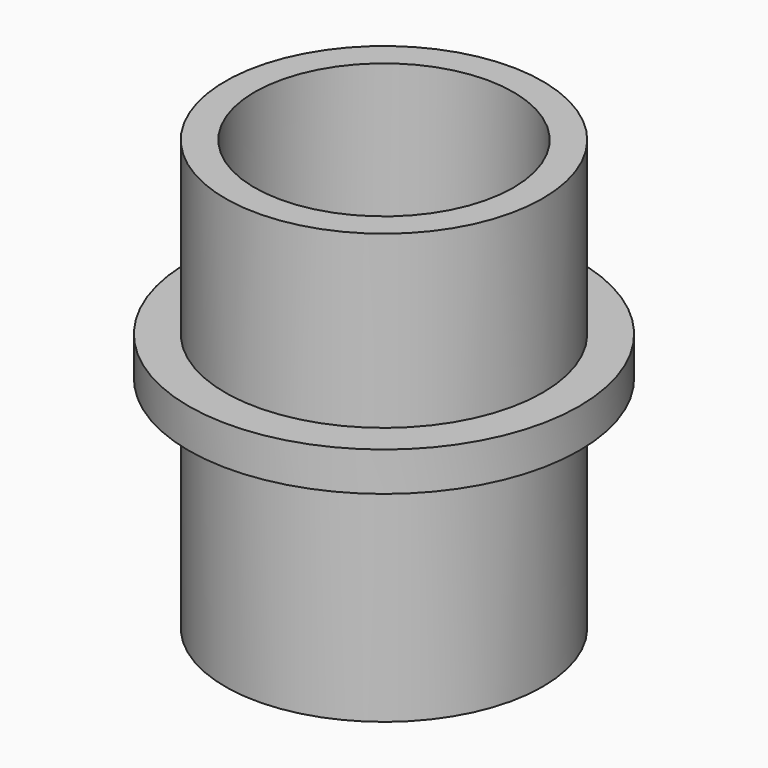
from build123d import *

# Parameters (mm, degrees)
F0_R     = 6.5
F1_DEPTH = 9
F2_R     = 8
F3_DEPTH = 1.6
F4_R     = 6.5
F5_DEPTH = 7
F6_T     = 1.2


# Not quite as in the source:
# - a shell that OpenCascade refuses in one call is made with other operations: the cavity is built on its own and cut out


with BuildPart() as f1:
    # F0 (on Top) → F1 (new body)
    with BuildSketch(Plane.XY):
        Circle(F0_R)
    extrude(amount=F1_DEPTH)

    # F2 (on face) → F3 (join)
    with BuildSketch(Plane.XY.offset(9)):
        Circle(F2_R)
    extrude(amount=F3_DEPTH)

    # F4 (on face) → F5 (join)
    with BuildSketch(Plane.XY.offset(10.6)):
        Circle(F4_R)
    extrude(amount=F5_DEPTH)

    # F6: shell of thickness 1.2, made by hand


with BuildPart() as f6_core1:
    # F6_t2: copy of F1
    add(f1.part)

    # the walls: a layer under each face that stays
    f6_faces = [f6_core1.faces().sort_by_distance(p)[0] for p in [
        (-8, 0, 9.8),
        (-5.3333333333, -5.3333333333, 9),
        (-5.3333333333, -5.3333333333, 10.6),
        (-6.5, 0, 4.5),
        (-6.5, 0, 14.1),
        (0, 0, 0),
    ]]
    thicken(f6_faces, amount=-F6_T, mode=Mode.SUBTRACT)

    # F6_s3 → F6_t4 (revolve, cut)
    with BuildSketch(Plane.XZ):
        Polygon((6.512, 8.988), (6.5, 10.2), (5.3, 10.2), (5.3, 9), align=None)
    revolve(axis=Axis((0, 0, 9), (0, 0, 1)), mode=Mode.SUBTRACT)

    # F6_s5 → F6_t6 (revolve, cut)
    with BuildSketch(Plane.XZ):
        Polygon((6.512, 10.612), (6.5, 9.4), (5.3, 9.4), (5.3, 10.6), align=None)
    revolve(axis=Axis((0, 0, 10.6), (0, 0, 1)), mode=Mode.SUBTRACT)


with BuildPart() as f1_1:
    add(f1.part)

    # what is left inside the walls is the cavity
    f6_cavity = [f6_core1.part.solids().sort_by_distance(p)[0] for p in [
        (-5.288, 0, 12.133333),
    ]]
    add(f6_cavity, mode=Mode.SUBTRACT)


solid = f1_1.part
